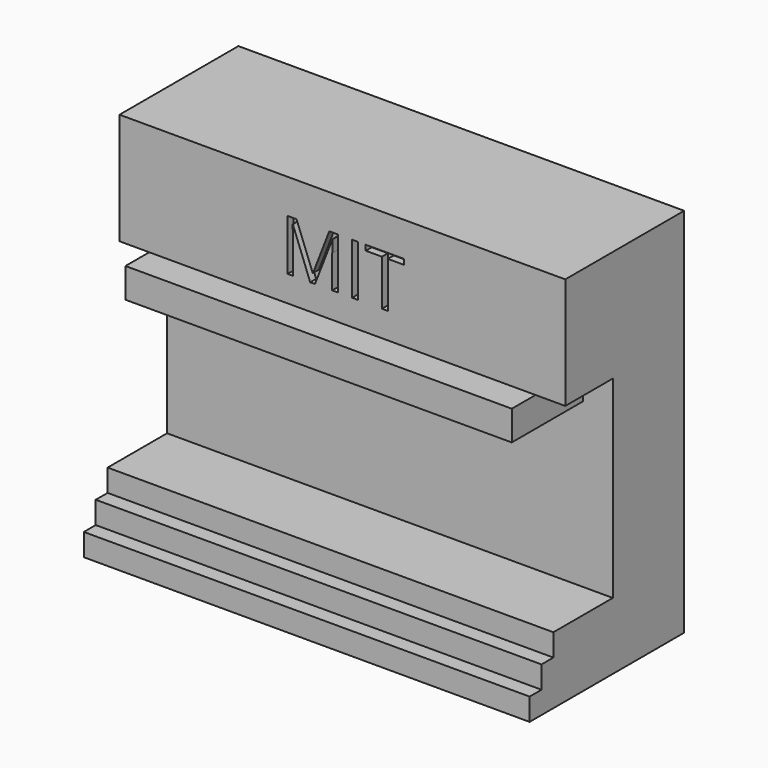
from build123d import *

# Parameters (mm, degrees)
F0_W          = 76.2
F0_H          = 25.4
F1_DEPTH      = 63.5
F2_W          = 76.2
F2_H          = 33.02
F3_DEPTH      = 10.16
F4_W          = 76.2
F4_H          = 3.81
F5_DEPTH      = 2.54
F6_W          = 76.2
F6_H          = 3.81
F7_DEPTH      = 5.08
F9_W          = 66.04
F9_H          = 5.08
F10_DEPTH     = 15.24
F8_W          = 76.2
F8_H          = 3.81
F11_DEPTH     = 7.62
F12_TEXT_SIZE = 12.2339412984
F13_DEPTH     = 1.27


# Not quite as in the source:
# - Text() gives the source's letters only with a copy of the font that has no kerning and outlines rounded to 1/6400 em; it was checked with that copy


with BuildPart() as f1:
    # F0 (on Top) → F1 (new body)
    with BuildSketch(Plane.XY):
        Rectangle(F0_W, F0_H)
    extrude(amount=F1_DEPTH)

    # F2 (on face) → F3 (cut)
    with BuildSketch(Plane.XZ.offset(12.7)):
        with Locations((0, 27.94)):
            Rectangle(F2_W, F2_H)
    extrude(amount=-F3_DEPTH, mode=Mode.SUBTRACT)

    # F4 (on face) → F5 (join)
    with BuildSketch(Plane.XZ.offset(12.7)):
        with Locations((0, 9.525)):
            Rectangle(F4_W, F4_H)
    extrude(amount=F5_DEPTH)

    # F6 (on face) → F7 (join)
    with BuildSketch(Plane.XZ.offset(12.7)):
        with Locations((0, 5.715)):
            Rectangle(F6_W, F6_H)
    extrude(amount=F7_DEPTH)

    # F9 (on face) → F10 (join)
    with BuildSketch(Plane.XZ.offset(2.54)):
        with Locations((0, 41.91)):
            Rectangle(F9_W, F9_H)
    extrude(amount=F10_DEPTH)

    # F8 (on face) → F11 (join)
    with BuildSketch(Plane.XZ.offset(12.7)):
        with Locations((0, 1.905)):
            Rectangle(F8_W, F8_H)
    extrude(amount=F11_DEPTH)

    # F12 (on face) → F13 (cut)
    with BuildSketch(Plane.XZ.offset(12.7)):
        with Locations((-10.5701251887, 48.886846751)):
            Text('MIT', F12_TEXT_SIZE, font='Open Sans', text_align=(TextAlign.LEFT, TextAlign.BOTTOM))
    extrude(amount=-F13_DEPTH, mode=Mode.SUBTRACT)


solid = f1.part
